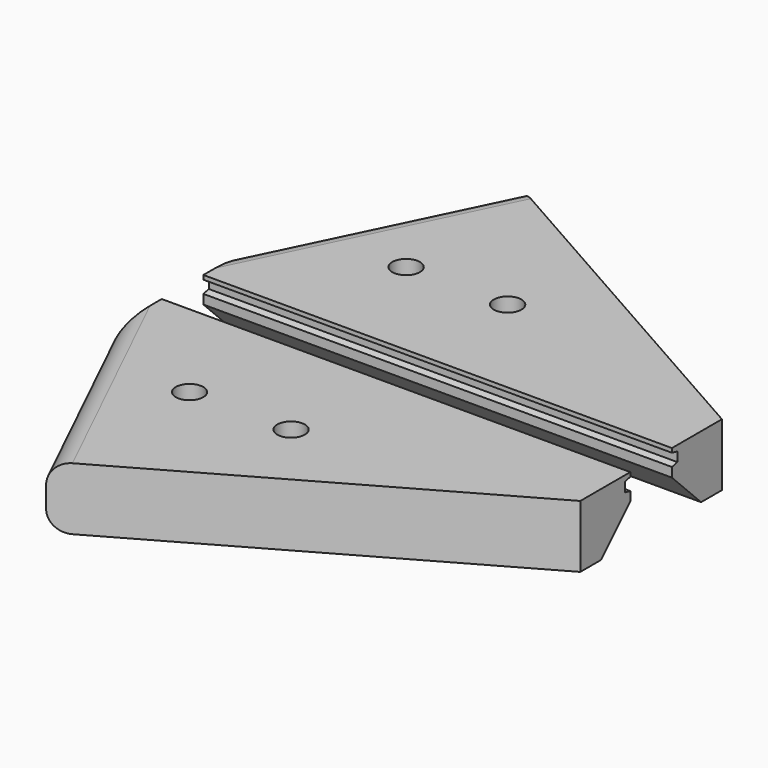
from build123d import *

# Parameters (mm, degrees)
F2_DEPTH         = 12
F3_D             = 5.3
F3_CBORE_D       = 9.75
F3_CBORE_DEPTH   = 3.2
F3_2_D           = 5.3
F3_2_CBORE_D     = 9.75
F3_2_CBORE_DEPTH = 3.2
F5_DEPTH         = 58.1081982567
F5_DEPTH_BACK    = 31.8938017433
F6_R             = 4
F6_2_R           = 4
F7_T1_DEPTH      = 126.0035618315
F7_2_T1_DEPTH    = 126.0035618315


# Not quite as in the source:
# - a fillet or chamfer that OpenCascade refuses, or shapes differently, is made with other operations: its cross-section is extruded or revolved along the edge and cut away or added
# - a feature names something its author has since deleted; it is built from what else it names


with BuildPart() as f2:
    # F1 (on Top) → F2 (new body)
    with BuildSketch(Plane.XY):
        Polygon((-31.8928017433, 17), (-31.8928017433, 5), (58.1071982567, 5), (58.1071982567, 17), (-12.5075216938, 56.9939360137), align=None)
    extrude(amount=F2_DEPTH)

    # F3 (through all)
    with Locations(Plane(origin=(0, 0, 0), x_dir=(1, 0, 0), z_dir=(0, 0, -1))):
        with Locations((-9.75, -26), (9.75, -26), (-9.75, 26), (9.75, 26)):
            CounterBoreHole(F3_D / 2, F3_CBORE_D / 2, F3_CBORE_DEPTH)


with BuildPart() as f2b:
    # F1 (on Top) → F2, piece 2 (new body)
    with BuildSketch(Plane.XY):
        Polygon((58.1071982567, -17), (58.1071982567, -5), (-31.8928017433, -5), (-31.8928017433, -17), (-12.5075216938, -56.9939360137), align=None)
    extrude(amount=F2_DEPTH)

    # F3#2 (through all)
    with Locations(Plane(origin=(0, 0, 0), x_dir=(1, 0, 0), z_dir=(0, 0, -1))):
        with Locations((-9.75, -26), (9.75, -26), (-9.75, 26), (9.75, 26)):
            CounterBoreHole(F3_2_D / 2, F3_2_CBORE_D / 2, F3_2_CBORE_DEPTH)


with BuildPart() as f5_tool:
    # F4 (on Right) → F5 (new body, two sides)
    with BuildSketch(Plane.YZ) as f5_sk:
        Polygon((-6.3, 10.9), (-6.3, 9.1), (-5, 8.8), (-5, 11.2), align=None)
        Polygon((6.3, 9.1), (6.3, 10.9), (5, 11.2), (5, 8.8), align=None)
    extrude(amount=F5_DEPTH)
    extrude(f5_sk.sketch, amount=-F5_DEPTH_BACK)


with BuildPart() as f2_1:
    add(f2.part)

    # F5: cut by f5_tool
    add(f5_tool.part, mode=Mode.SUBTRACT)

    # F6
    f6_edges = [f2_1.edges().sort_by_distance(p)[0] for p in [
        (-22.200162, 36.996968, 12),
        (-22.200162, 36.996968, 0),
    ]]
    fillet(f6_edges, radius=F6_R)

    # F7: chamfer of 7 on 1 edges, made by hand

    # F7_s2 → F7_t1 (cut)
    with BuildSketch(Plane.YZ.offset(-49.894582659)):
        Polygon((12, 0), (5, 7), (5, 0), align=None)
    extrude(amount=F7_T1_DEPTH, mode=Mode.SUBTRACT)


with BuildPart() as f2b_1:
    add(f2b.part)

    # F5: cut by f5_tool
    add(f5_tool.part, mode=Mode.SUBTRACT)

    # F6#2
    f6_2_edges = [f2b_1.edges().sort_by_distance(p)[0] for p in [
        (-22.200162, -36.996968, 0),
        (-22.200162, -36.996968, 12),
    ]]
    fillet(f6_2_edges, radius=F6_2_R)

    # F7#2: chamfer of 7 on 1 edges, made by hand

    # F7_2_s2 → F7_2_t1 (cut)
    with BuildSketch(Plane.YZ.offset(-49.894582659)):
        Polygon((-12, 0), (-5, 7), (-5, 0), align=None)
    extrude(amount=F7_2_T1_DEPTH, mode=Mode.SUBTRACT)


solid = Compound([f2_1.part, f2b_1.part])
